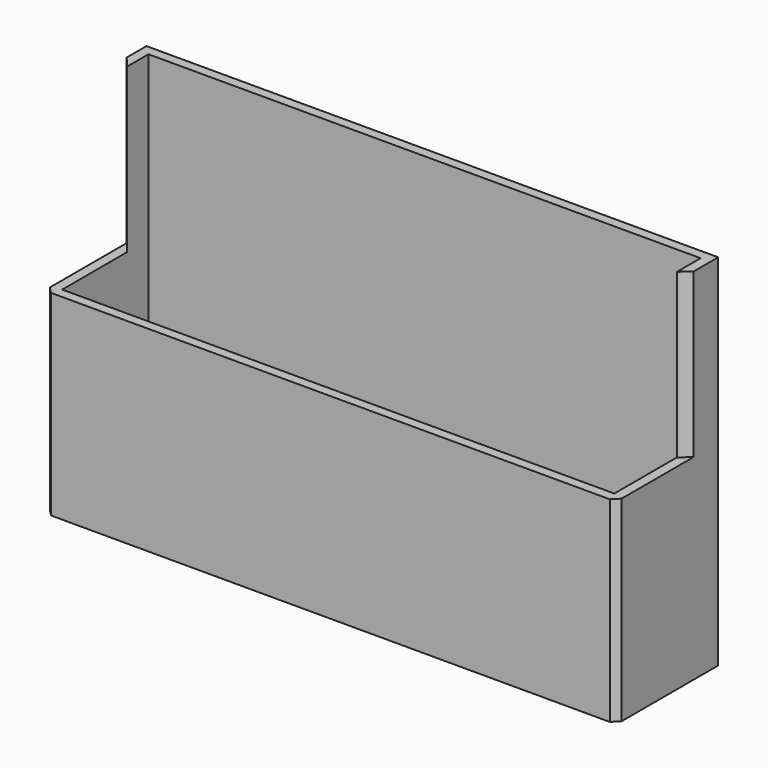
from build123d import *

# Parameters (mm, degrees)
F0_W        = 87.5
F0_H        = 19.5
F0_W_2      = 84.5
F0_H_2      = 16.5
F1_DEPTH    = 30
F2_DEPTH    = 3
F3_SIZE     = 1
F5_DEPTH    = 25
F6_DEPTH    = 25
F7_T1_DEPTH = 40.3581649162


# Not quite as in the source:
# - a fillet or chamfer that OpenCascade refuses, or shapes differently, is made with other operations: its cross-section is extruded or revolved along the edge and cut away or added


with BuildPart() as f1:
    # F0 (on Top) → F1 (new body)
    with BuildSketch(Plane.XY):
        Rectangle(F0_W, F0_H)
        Rectangle(F0_W_2, F0_H_2, mode=Mode.SUBTRACT)
    extrude(amount=F1_DEPTH)

    # F0 (on Top) → F2 (join)
    with BuildSketch(Plane.XY):
        Rectangle(F0_W_2, F0_H_2)
    extrude(amount=F2_DEPTH)

    # F3
    f3_edges = [f1.edges().sort_by_distance(p)[0] for p in [
        (-43.75, -9.75, 15),
        (43.75, -9.75, 15),
    ]]
    chamfer(f3_edges, length=F3_SIZE)

    # F4 (on face) → F5 (join)
    with BuildSketch(Plane.XY.offset(30)):
        Polygon((-43.75, 9.75), (-43.75, 0), (-42.25, 0), (-42.25, 8.25), (42.25, 8.25), (42.25, 0), (43.75, 0), (43.75, 9.75), align=None)
    extrude(amount=F5_DEPTH)

    # F4 (on face) → F6 (cut)
    with BuildSketch(Plane.XY.offset(30)):
        Polygon((50.0001870096, 0), (-45.6664785743, 0), (-48.1942594051, -2.8349049389), (-42.25, -20.2376823872), (42.25, -19.071014598), align=None)
    extrude(amount=F6_DEPTH, mode=Mode.SUBTRACT)

    # F7: chamfer of 5 x 5.958767963 on 2 edges, made by hand

    # F7_s2 → F7_t1 (cut)
    with BuildSketch(Plane.XY.offset(30)):
        Polygon((-43.75, 5.958767963), (-38.75, 0), (-43.75, 0), align=None)
        Polygon((43.75, 5), (37.791232037, 0), (43.75, 0), align=None)
    extrude(amount=F7_T1_DEPTH, mode=Mode.SUBTRACT)


solid = f1.part
